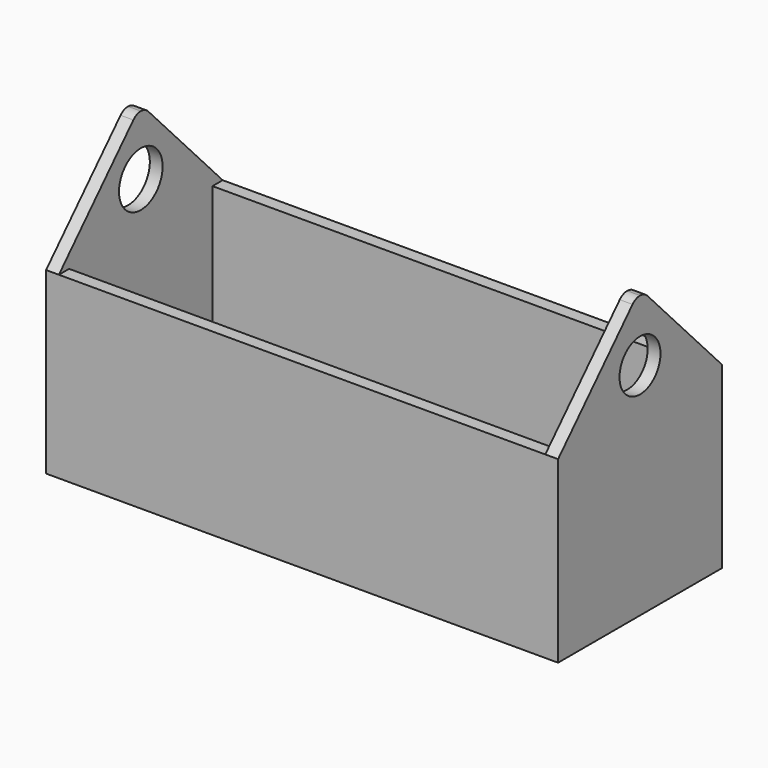
from build123d import *

# Parameters (mm, degrees)
F0_W      = 254
F0_H      = 101.6
F1_DEPTH  = 88.9
F4_DEPTH  = 6.35
F2_W      = 241.3
F2_H      = 88.9
F8_DEPTH  = 82.55
F9_R      = 12.7
F10_DEPTH = 25.4
F11_R     = 13.5154213428
F12_DEPTH = 25.4


with BuildPart() as f1:
    # F0 (on Top) → F1 (new body)
    with BuildSketch(Plane.XY):
        with Locations((77.3512227356, 27.0002914594)):
            Rectangle(F0_W, F0_H)
    extrude(amount=F1_DEPTH)

    # F3 (on face) → F4 (join)
    with BuildSketch(Plane.YZ.offset(204.3512227356)):
        with BuildLine():
            Line((22.3877730248, 137.7143067824), (-23.7997085406, 88.9))
            Line((-23.7997085406, 88.9), (27.0002914594, 88.9))
            Line((27.0002914594, 88.9), (27.0002914594, 139.7))
            ThreePointArc((27.0002914594, 139.7), (24.489399991, 139.1824886656), (22.3877730248, 137.7143067824))
        make_face()
        with BuildLine():
            Line((27.0002914594, 139.7), (27.0002914594, 88.9))
            Line((27.0002914594, 88.9), (77.8002914594, 88.9))
            Line((77.8002914594, 88.9), (31.6128098939, 137.7143067824))
            ThreePointArc((31.6128098939, 137.7143067824), (29.5111829277, 139.1824886656), (27.0002914594, 139.7))
        make_face()
    extrude(amount=-F4_DEPTH)

    # F7: F1 across plane


with BuildPart() as f1_1:
    add(f1.part)
    add(f1.part.mirror(Plane(origin=(77.3512227356, 27.0002914594, 88.9), x_dir=(0, 1, 0), z_dir=(1, 0, 0))))

    # F2 (on face) → F8 (cut)
    with BuildSketch(Plane.XY.offset(88.9)):
        with Locations((77.3512227356, 27.0002914594)):
            Rectangle(F2_W, F2_H)
    extrude(amount=-F8_DEPTH, mode=Mode.SUBTRACT)

    # F9 (on face) → F10 (cut)
    with BuildSketch(Plane.YZ.offset(204.3512227356)):
        with Locations((27.0002914594, 109.2127263546)):
            Circle(F9_R)
    extrude(amount=-F10_DEPTH, mode=Mode.SUBTRACT)

    # F11 (on face) → F12 (cut)
    with BuildSketch(Plane(origin=(-49.6487772644, 0, 0), x_dir=(0, -1, 0), z_dir=(-1, 0, 0))):
        with Locations((-27.0002914594, 110.0281476974)):
            Circle(F11_R)
    extrude(amount=-F12_DEPTH, mode=Mode.SUBTRACT)


solid = f1_1.part
